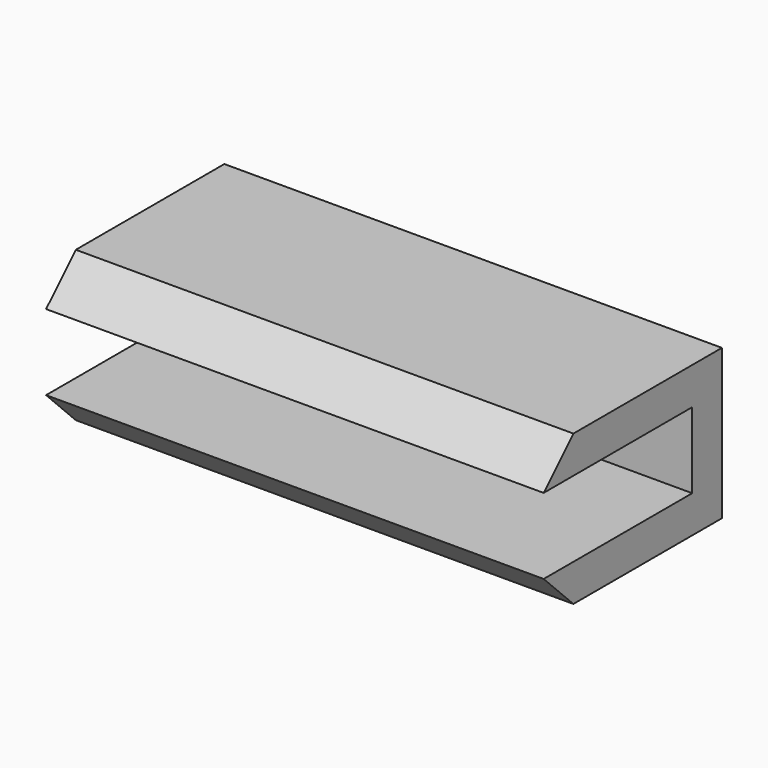
from build123d import *

# Parameters (mm, degrees)
F0_W     = 67
F0_H     = 5
F1_DEPTH = 10.2
F2_W     = 67
F2_H     = 25
F2_H_2   = 5
F3_DEPTH = 5
F4_SIZE  = 4.99999
F5_W     = 67
F5_H     = 5
F5_H_2   = 25
F6_DEPTH = 5
F7_SIZE  = 4.99999


# Not quite as in the source:
# - a fillet or chamfer is up to 0.001 mm smaller than in the source, because OpenCascade refuses the exact size


with BuildPart() as f1:
    # F0 (on Top) → F1 (new body)
    with BuildSketch(Plane.XY):
        Rectangle(F0_W, F0_H)
    extrude(amount=F1_DEPTH)

    # F2 (on face) → F3 (join)
    with BuildSketch(Plane.XY.offset(10.2)):
        with Locations((0, -15)):
            Rectangle(F2_W, F2_H)
        Rectangle(F2_W, F2_H_2)
    extrude(amount=F3_DEPTH)

    # F4 (size 5 in the source; OpenCascade refuses exactly that, so slightly less here)
    f4_edges = [f1.edges().sort_by_distance(p)[0] for p in [
        (0, -27.5, 15.2),
    ]]
    chamfer(f4_edges, length=F4_SIZE)

    # F5 (on face) → F6 (join)
    with BuildSketch(Plane(origin=(0, 0, 0), x_dir=(1, 0, 0), z_dir=(0, 0, -1))):
        Rectangle(F5_W, F5_H)
        with Locations((0, 15)):
            Rectangle(F5_W, F5_H_2)
    extrude(amount=F6_DEPTH)

    # F7 (size 5 in the source; OpenCascade refuses exactly that, so slightly less here)
    f7_edges = [f1.edges().sort_by_distance(p)[0] for p in [
        (0, -27.5, -5),
    ]]
    chamfer(f7_edges, length=F7_SIZE)


solid = f1.part
